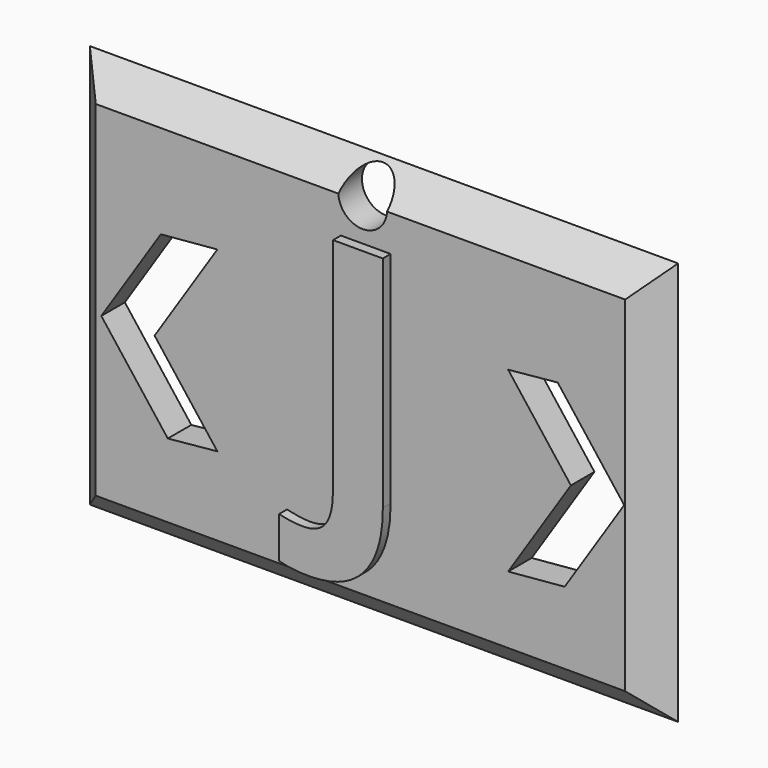
from build123d import *

# Parameters (mm, degrees)
F0_W         = 78.6983631551
F0_H         = 54.7973793
F0_R         = 3.1476833793
F1_DEPTH     = 3.81
F0_TEXT_SIZE = 42.5424604364
F2_DEPTH     = 5.08
F3_T1_DEPTH  = 80.9256784577
F3_T3_DEPTH  = 104.8266623129


# Not quite as in the source:
# - a fillet or chamfer that OpenCascade refuses, or shapes differently, is made with other operations: its cross-section is extruded or revolved along the edge and cut away or added
# - Text() gives the source's letters only with a copy of the font that has no kerning and outlines rounded to 1/6400 em; it was checked with that copy


with BuildPart() as f1:
    # F0 (on Front) → F1 (new body)
    with BuildSketch(Plane.XZ):
        with Locations((-0.2914760262, 1.6031144187)):
            Rectangle(F0_W, F0_H)
        Polygon((-25.2329215557, -11.1686556562), (-33.842036543, 0), (-26.1391318392, 11.8119003194), (-18.8194342679, 12.458750179), (-26.9441697264, 0), (-18.8194342679, -10.5473195323), align=None, mode=Mode.SUBTRACT)
        with BuildLine():
            add(Edge.make_bspline(
                [(1.1875378422, -17.2739692017), (-1.2420354843, -20.0591709084), (-6.0014732456, -20.0591709084)],
                knots=[0, 0, 0, 1, 1, 1], degree=2))
            add(Edge.make_bspline(
                [(-6.0014732456, -20.0591709084), (-8.181774343, -20.0591709084), (-9.8037056471, -19.6005100068)],
                knots=[0, 0, 0, 1, 1, 1], degree=2))
            Line((-9.8037056471, -19.6005100068), (-9.8037056471, -14.2428188956))
            add(Edge.make_bspline(
                [(-9.8037056471, -14.2428188956), (-8.1418907863, -14.6549489811), (-6.772555341, -14.6549489811)],
                knots=[0, 0, 0, 1, 1, 1], degree=2))
            add(Edge.make_bspline(
                [(-6.772555341, -14.6549489811), (-4.6520795787, -14.6549489811), (-3.7380814052, -13.3354679816)],
                knots=[0, 0, 0, 1, 1, 1], degree=2))
            add(Edge.make_bspline(
                [(-3.7380814052, -13.3354679816), (-2.8240832318, -12.0159869821), (-2.8240832318, -9.2108434971)],
                knots=[0, 0, 0, 1, 1, 1], degree=2))
            Line((-2.8240832318, -9.2108434971), (-2.8240832318, 19.2460741792))
            Line((-2.8240832318, 19.2460741792), (3.6171111687, 19.2460741792))
            Line((3.6171111687, 19.2460741792), (3.6171111687, -9.1709599405))
            add(Edge.make_bspline(
                [(3.6171111687, -9.1709599405), (3.6171111687, -14.488767495), (1.1875378422, -17.2739692017)],
                knots=[0, 0, 0, 1, 1, 1], degree=2))
        make_face(mode=Mode.SUBTRACT)
        Polygon((25.2420099994, 11.6243917969), (33.8511249866, 0.4557361407), (26.1482202828, -11.3561641787), (18.8285227115, -12.0030140383), (26.9532581701, 0.4557361407), (18.8285227115, 11.003055673), align=None, mode=Mode.SUBTRACT)
        with Locations((0, 24.0467209369)):
            Circle(F0_R, mode=Mode.SUBTRACT)
    extrude(amount=F1_DEPTH)

    # F0 (on Front) → F2 (join)
    with BuildSketch(Plane.XZ):
        with Locations((-6.6462574116, -11.1252542168)):
            Text('J', F0_TEXT_SIZE, font='Open Sans', font_style=FontStyle.BOLD, text_align=(TextAlign.LEFT, TextAlign.BOTTOM))
    extrude(amount=F2_DEPTH)

    # F3: chamfer of 5.08 on 4 edges, made by hand

    # F3_s2 → F3_t1 (cut)
    with BuildSketch(Plane.XY.offset(-38.8597248102)):
        Polygon((-34.5606576037, -3.81), (-39.6406576037, 1.27), (-39.6406576037, -3.81), align=None)
        Polygon((39.0577055514, 1.27), (33.9777055514, -3.81), (39.0577055514, -3.81), align=None)
    extrude(amount=F3_T1_DEPTH, mode=Mode.SUBTRACT)

    # F3_s4 → F3_t3 (cut)
    with BuildSketch(Plane.YZ.offset(-52.7048071826)):
        Polygon((1.27, 29.0018040687), (-3.81, 23.9218040687), (-3.81, 29.0018040687), align=None)
        Polygon((1.27, -25.7955752313), (-3.81, -20.7155752313), (-3.81, -25.7955752313), align=None)
    extrude(amount=F3_T3_DEPTH, mode=Mode.SUBTRACT)


solid = f1.part
